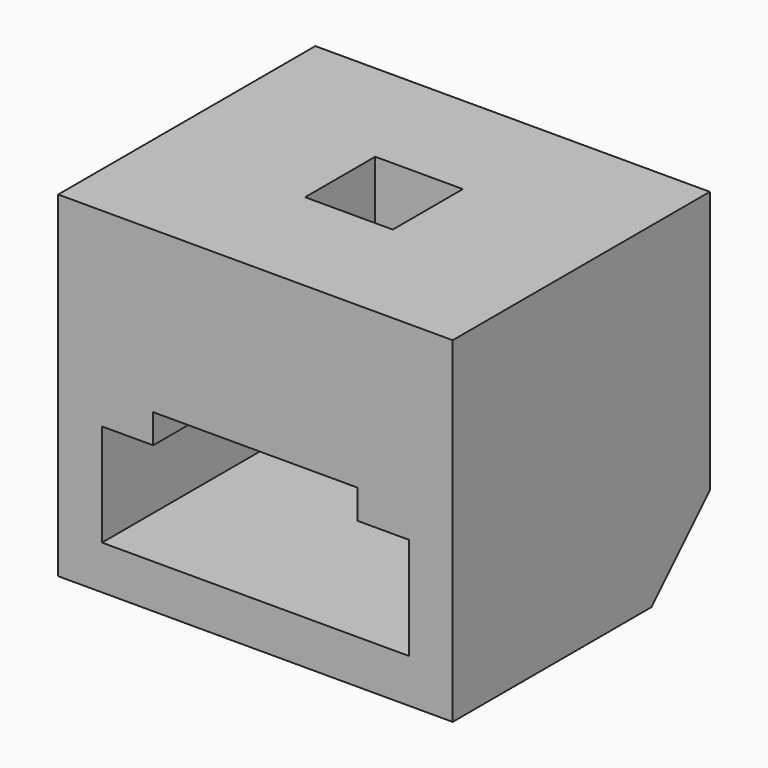
from build123d import *

# Parameters (mm, degrees)
F0_W         = 27
F0_H         = 22
F1_DEPTH     = 20
F2_W         = 21
F2_H         = 21
F3_DEPTH     = 6
F5_DEPTH     = 2
F7_DEPTH     = 20
F8_DEPTH     = 6
F9_W         = 27
F9_H         = 22
F10_DEPTH    = 3
F11_T1_DEPTH = 52.7168298797
F12_DEPTH    = 1


# Not quite as in the source:
# - a fillet or chamfer that OpenCascade refuses, or shapes differently, is made with other operations: its cross-section is extruded or revolved along the edge and cut away or added


with BuildPart() as f1:
    # F0 (on Top) → F1 (new body)
    with BuildSketch(Plane.XY):
        Rectangle(F0_W, F0_H)
    extrude(amount=F1_DEPTH)

    # F2 (on face) → F3 (cut)
    with BuildSketch(Plane(origin=(0, 0, 0), x_dir=(1, 0, 0), z_dir=(0, 0, -1))):
        with Locations((0, 0.5)):
            Rectangle(F2_W, F2_H)
    extrude(amount=-F3_DEPTH, mode=Mode.SUBTRACT)

    # F4 (on face) → F5 (cut)
    with BuildSketch(Plane(origin=(0, 0, 6), x_dir=(1, 0, 0), z_dir=(0, 0, -1))):
        Polygon((0, 11), (-7, 11), (-7, -11), (7, -11), (7, 11), align=None)
    extrude(amount=-F5_DEPTH, mode=Mode.SUBTRACT)

    # F6 (on face) → F7 (cut)
    with BuildSketch(Plane.XY.offset(20)):
        Polygon((0, -3), (3, -3), (3, 3), (-3, 3), (-3, -3), align=None)
    extrude(amount=-F7_DEPTH, mode=Mode.SUBTRACT)

    # F8 (cut): a face of the model
    f8_faces = [f1.faces().sort_by_distance(p)[0] for p in [
        (0, 10.5, 6),
    ]]
    extrude(f8_faces, amount=-F8_DEPTH, mode=Mode.SUBTRACT)

    # F9 (on face) → F10 (join)
    with BuildSketch(Plane(origin=(0, 0, 0), x_dir=(1, 0, 0), z_dir=(0, 0, -1))):
        Rectangle(F9_W, F9_H)
    extrude(amount=F10_DEPTH)

    # F11: chamfer of 5 on 1 edges, made by hand

    # F11_s2 → F11_t1 (cut)
    with BuildSketch(Plane.YZ.offset(-26.3584149398)):
        Polygon((11, 2), (6, -3), (11, -3), align=None)
    extrude(amount=F11_T1_DEPTH, mode=Mode.SUBTRACT)

    # F12 (cut): faces of the model
    f12_faces = [f1.faces().sort_by_distance(p)[0] for p in [
        (8.75, -0.5, 6),
        (-6.7392319038, 0, 8),
        (-8.75, -0.5, 6),
    ]]
    extrude(f12_faces, amount=-F12_DEPTH, mode=Mode.SUBTRACT)


solid = f1.part
